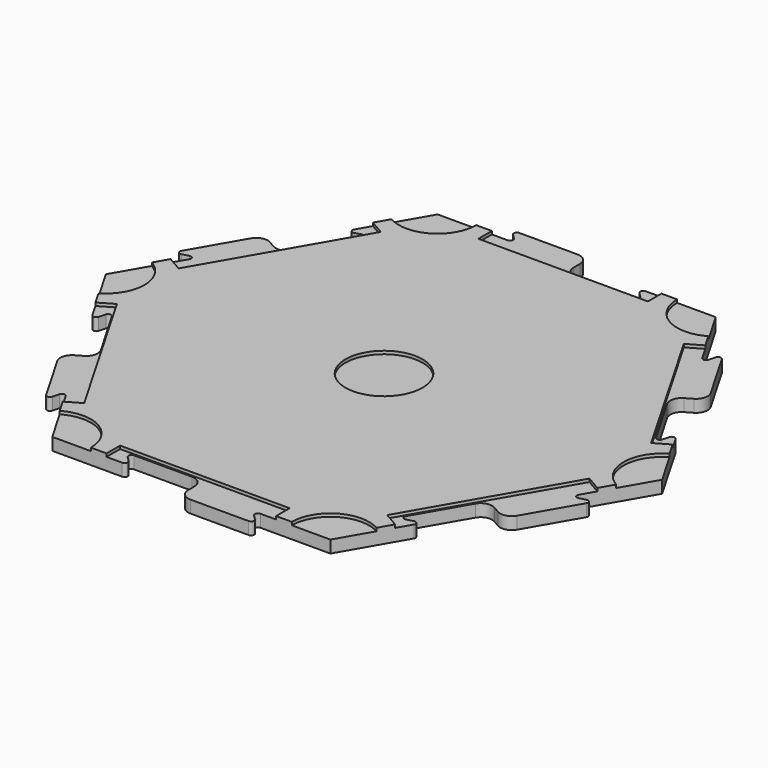
from build123d import *

# Parameters (mm, degrees)
F1_DEPTH = 2.54
F2_COUNT = 6
F4_R     = 6.35
F5_DEPTH = 0.508


# Not quite as in the source:
# - a feature names something its author has since deleted; it is built from what else it names


with BuildPart() as f1:
    # F0 (on Top) → F1 (new body)
    with BuildSketch(Plane.XY):
        with BuildLine():
            Line((11.3864204897, -39.6875), (22.9135888085, -39.6875))
            Line((22.9135888085, -39.6875), (0, 0))
            Line((0, 0), (-22.9135888085, -39.6875))
            Line((-22.9135888085, -39.6875), (-11.3864204897, -39.6875))
            ThreePointArc((-11.3864204897, -39.6875), (-10.9170896872, -39.3739031836), (-11.0272102448, -38.8202897552))
            Line((-11.0272102448, -38.8202897552), (-11.8327897552, -38.0147102448))
            ThreePointArc((-11.8327897552, -38.0147102448), (-11.9429103128, -37.4610968164), (-11.4735795103, -37.1475))
            Line((-11.4735795103, -37.1475), (-1.905, -37.1475))
            ThreePointArc((-1.905, -37.1475), (-0.5579615818, -37.7054615818), (0, -39.0525))
            Line((0, -39.0525), (0, -39.6875))
            Line((0, -39.6875), (11.3864204897, -39.6875))
        make_face()
        with BuildLine():
            ThreePointArc((11.0272102448, -40.5547102448), (10.9170896872, -40.0010968164), (11.3864204897, -39.6875))
            Line((11.3864204897, -39.6875), (0, -39.6875))
            Line((0, -39.6875), (0, -40.3225))
            ThreePointArc((0, -40.3225), (0.5579615818, -41.6695384182), (1.905, -42.2275))
            Line((1.905, -42.2275), (11.4735795103, -42.2275))
            ThreePointArc((11.4735795103, -42.2275), (11.9429103128, -41.9139031836), (11.8327897552, -41.3602897552))
            Line((11.8327897552, -41.3602897552), (11.0272102448, -40.5547102448))
        make_face()
    extrude(amount=F1_DEPTH)


with BuildPart() as f2_1:
    # F2: instance of F1
    add(f1.part.rotate(Axis((0, 0, 1.27), (0, 0, -1)), 1 * 360 / F2_COUNT))


with BuildPart() as f2_2:
    # F2: instance of F1
    add(f1.part.rotate(Axis((0, 0, 1.27), (0, 0, -1)), 2 * 360 / F2_COUNT))


with BuildPart() as f2_3:
    # F2: instance of F1
    add(f1.part.rotate(Axis((0, 0, 1.27), (0, 0, -1)), 3 * 360 / F2_COUNT))


with BuildPart() as f2_4:
    # F2: instance of F1
    add(f1.part.rotate(Axis((0, 0, 1.27), (0, 0, -1)), 4 * 360 / F2_COUNT))


with BuildPart() as f2_5:
    # F2: instance of F1
    add(f1.part.rotate(Axis((0, 0, 1.27), (0, 0, -1)), 5 * 360 / F2_COUNT))


with BuildPart() as f1_1:
    add(f1.part)

    # F3: union F2_1, F2_2, F2_3, F2_4, F2_5
    add(f2_1.part)
    add(f2_2.part)
    add(f2_3.part)
    add(f2_4.part)
    add(f2_5.part)

    # F4 (on face) → F5 (cut)
    with BuildSketch(Plane.XY.offset(2.54)):
        with BuildLine():
            Line((13.97, -36.8935), (-13.97, -36.8935))
            Line((-13.97, -36.8935), (-13.97, -39.6875))
            Line((-13.97, -39.6875), (-11.3864204897, -39.6875))
            ThreePointArc((-11.3864204897, -39.6875), (-10.9170896872, -39.3739031836), (-11.0272102448, -38.8202897552))
            Line((-11.0272102448, -38.8202897552), (-11.8327897552, -38.0147102448))
            ThreePointArc((-11.8327897552, -38.0147102448), (-11.9429103128, -37.4610968164), (-11.4735795103, -37.1475))
            Line((-11.4735795103, -37.1475), (-1.905, -37.1475))
            ThreePointArc((-1.905, -37.1475), (-0.5579615818, -37.7054615818), (0, -39.0525))
            Line((0, -39.0525), (0, -40.3225))
            ThreePointArc((0, -40.3225), (0.5579615818, -41.6695384182), (1.905, -42.2275))
            Line((1.905, -42.2275), (11.4735795103, -42.2275))
            ThreePointArc((11.4735795103, -42.2275), (11.9429103128, -41.9139031836), (11.8327897552, -41.3602897552))
            Line((11.8327897552, -41.3602897552), (11.0272102448, -40.5547102448))
            ThreePointArc((11.0272102448, -40.5547102448), (10.9170896872, -40.0010968164), (11.3864204897, -39.6875))
            Line((11.3864204897, -39.6875), (13.97, -39.6875))
            Line((13.97, -39.6875), (13.97, -36.8935))
        make_face()
        with BuildLine():
            Line((-22.9135888085, -39.6875), (-16.5635888085, -39.6875))
            ThreePointArc((-16.5635888085, -39.6875), (-19.7385888085, -34.188238686), (-26.0885888085, -34.188238686))
            Line((-26.0885888085, -34.188238686), (-22.9135888085, -39.6875))
        make_face()
        with BuildLine():
            ThreePointArc((26.0885888085, -34.188238686), (19.7385888085, -34.188238686), (16.5635888085, -39.6875))
            Line((16.5635888085, -39.6875), (22.9135888085, -39.6875))
            Line((22.9135888085, -39.6875), (26.0885888085, -34.188238686))
        make_face()
        with BuildLine():
            Line((-28.6771729679, -29.7046794022), (-27.3853832127, -31.9421248909))
            Line((-27.3853832127, -31.9421248909), (-24.9657082345, -30.5451248909))
            Line((-24.9657082345, -30.5451248909), (-38.9357082345, -6.3483751091))
            Line((-38.9357082345, -6.3483751091), (-41.3553832127, -7.7453751091))
            Line((-41.3553832127, -7.7453751091), (-40.0635934575, -9.9828205978))
            ThreePointArc((-40.0635934575, -9.9828205978), (-39.5573452468, -10.2324745873), (-39.1329622327, -9.8603006727))
            Line((-39.1329622327, -9.8603006727), (-38.8380996671, -8.7598585968))
            ThreePointArc((-38.8380996671, -8.7598585968), (-38.413716653, -8.3876846821), (-37.9074684422, -8.6373386717))
            Line((-37.9074684422, -8.6373386717), (-33.1231786871, -16.9239716058))
            ThreePointArc((-33.1231786871, -16.9239716058), (-32.9328683822, -18.3695218867), (-33.8204570813, -19.52625))
            Line((-33.8204570813, -19.52625), (-34.9203093441, -20.16125))
            ThreePointArc((-34.9203093441, -20.16125), (-35.8078980432, -21.3179781133), (-35.6175877383, -22.7635283942))
            Line((-35.6175877383, -22.7635283942), (-30.8332979832, -31.0501613283))
            ThreePointArc((-30.8332979832, -31.0501613283), (-30.3270497724, -31.2998153179), (-29.9026667583, -30.9276414032))
            Line((-29.9026667583, -30.9276414032), (-29.6078041927, -29.8271993273))
            ThreePointArc((-29.6078041927, -29.8271993273), (-29.1834211786, -29.4550254127), (-28.6771729679, -29.7046794022))
        make_face()
        with BuildLine():
            Line((24.9657082345, -30.5451248909), (27.3853832127, -31.9421248909))
            Line((27.3853832127, -31.9421248909), (28.6771729679, -29.7046794022))
            ThreePointArc((28.6771729679, -29.7046794022), (28.6402555596, -29.1414285963), (28.1057519878, -28.9599890825))
            Line((28.1057519878, -28.9599890825), (27.005309912, -29.254851648))
            ThreePointArc((27.005309912, -29.254851648), (26.4708063402, -29.0734121342), (26.4338889319, -28.5101613283))
            Line((26.4338889319, -28.5101613283), (31.2181786871, -20.2235283942))
            ThreePointArc((31.2181786871, -20.2235283942), (32.3749068004, -19.3359396951), (33.8204570813, -19.52625))
            Line((33.8204570813, -19.52625), (34.9203093441, -20.16125))
            ThreePointArc((34.9203093441, -20.16125), (36.365859625, -20.3515603049), (37.5225877383, -19.4639716058))
            Line((37.5225877383, -19.4639716058), (42.3068774935, -11.1773386717))
            ThreePointArc((42.3068774935, -11.1773386717), (42.2699600852, -10.6140878658), (41.7354565134, -10.432648352))
            Line((41.7354565134, -10.432648352), (40.6350144376, -10.7275109175))
            ThreePointArc((40.6350144376, -10.7275109175), (40.1005108658, -10.5460714037), (40.0635934575, -9.9828205978))
            Line((40.0635934575, -9.9828205978), (41.3553832127, -7.7453751091))
            Line((41.3553832127, -7.7453751091), (38.9357082345, -6.3483751091))
            Line((38.9357082345, -6.3483751091), (24.9657082345, -30.5451248909))
        make_face()
        with BuildLine():
            Line((-45.8271776169, 0), (-42.6521776169, -5.499261314))
            ThreePointArc((-42.6521776169, -5.499261314), (-40.3279163029, -3.175), (-39.4771776169, 0))
            ThreePointArc((-39.4771776169, 0), (-40.3279163029, 3.175), (-42.6521776169, 5.499261314))
            Line((-42.6521776169, 5.499261314), (-45.8271776169, 0))
        make_face()
        with BuildLine():
            ThreePointArc((42.6521776169, 5.499261314), (39.4771776169, 0), (42.6521776169, -5.499261314))
            Line((42.6521776169, -5.499261314), (45.8271776169, 0))
            Line((45.8271776169, 0), (42.6521776169, 5.499261314))
        make_face()
        with BuildLine():
            Line((-40.0635934575, 9.9828205978), (-41.3553832127, 7.7453751091))
            Line((-41.3553832127, 7.7453751091), (-38.9357082345, 6.3483751091))
            Line((-38.9357082345, 6.3483751091), (-24.9657082345, 30.5451248909))
            Line((-24.9657082345, 30.5451248909), (-27.3853832127, 31.9421248909))
            Line((-27.3853832127, 31.9421248909), (-28.6771729679, 29.7046794022))
            ThreePointArc((-28.6771729679, 29.7046794022), (-28.6402555596, 29.1414285963), (-28.1057519878, 28.9599890825))
            Line((-28.1057519878, 28.9599890825), (-27.005309912, 29.254851648))
            ThreePointArc((-27.005309912, 29.254851648), (-26.4708063402, 29.0734121342), (-26.4338889319, 28.5101613283))
            Line((-26.4338889319, 28.5101613283), (-31.2181786871, 20.2235283942))
            ThreePointArc((-31.2181786871, 20.2235283942), (-32.3749068004, 19.3359396951), (-33.8204570813, 19.52625))
            Line((-33.8204570813, 19.52625), (-34.9203093441, 20.16125))
            ThreePointArc((-34.9203093441, 20.16125), (-36.365859625, 20.3515603049), (-37.5225877383, 19.4639716058))
            Line((-37.5225877383, 19.4639716058), (-42.3068774935, 11.1773386717))
            ThreePointArc((-42.3068774935, 11.1773386717), (-42.2699600852, 10.6140878658), (-41.7354565134, 10.432648352))
            Line((-41.7354565134, 10.432648352), (-40.6350144376, 10.7275109175))
            ThreePointArc((-40.6350144376, 10.7275109175), (-40.1005108658, 10.5460714037), (-40.0635934575, 9.9828205978))
        make_face()
        with BuildLine():
            Line((38.9357082345, 6.3483751091), (41.3553832127, 7.7453751091))
            Line((41.3553832127, 7.7453751091), (40.0635934575, 9.9828205978))
            ThreePointArc((40.0635934575, 9.9828205978), (39.5573452468, 10.2324745873), (39.1329622327, 9.8603006727))
            Line((39.1329622327, 9.8603006727), (38.8380996671, 8.7598585968))
            ThreePointArc((38.8380996671, 8.7598585968), (38.413716653, 8.3876846821), (37.9074684422, 8.6373386717))
            Line((37.9074684422, 8.6373386717), (33.1231786871, 16.9239716058))
            ThreePointArc((33.1231786871, 16.9239716058), (32.9328683822, 18.3695218867), (33.8204570813, 19.52625))
            Line((33.8204570813, 19.52625), (34.9203093441, 20.16125))
            ThreePointArc((34.9203093441, 20.16125), (35.8078980432, 21.3179781133), (35.6175877383, 22.7635283942))
            Line((35.6175877383, 22.7635283942), (30.8332979832, 31.0501613283))
            ThreePointArc((30.8332979832, 31.0501613283), (30.3270497724, 31.2998153179), (29.9026667583, 30.9276414032))
            Line((29.9026667583, 30.9276414032), (29.6078041927, 29.8271993273))
            ThreePointArc((29.6078041927, 29.8271993273), (29.1834211786, 29.4550254127), (28.6771729679, 29.7046794022))
            Line((28.6771729679, 29.7046794022), (27.3853832127, 31.9421248909))
            Line((27.3853832127, 31.9421248909), (24.9657082345, 30.5451248909))
            Line((24.9657082345, 30.5451248909), (38.9357082345, 6.3483751091))
        make_face()
        with BuildLine():
            Line((-22.9135888085, 39.6875), (-26.0885888085, 34.188238686))
            ThreePointArc((-26.0885888085, 34.188238686), (-19.7385888085, 34.188238686), (-16.5635888085, 39.6875))
            Line((-16.5635888085, 39.6875), (-22.9135888085, 39.6875))
        make_face()
        with BuildLine():
            ThreePointArc((16.5635888085, 39.6875), (19.7385888085, 34.188238686), (26.0885888085, 34.188238686))
            Line((26.0885888085, 34.188238686), (22.9135888085, 39.6875))
            Line((22.9135888085, 39.6875), (16.5635888085, 39.6875))
        make_face()
        with BuildLine():
            Line((-11.3864204897, 39.6875), (-13.97, 39.6875))
            Line((-13.97, 39.6875), (-13.97, 36.8935))
            Line((-13.97, 36.8935), (13.97, 36.8935))
            Line((13.97, 36.8935), (13.97, 39.6875))
            Line((13.97, 39.6875), (11.3864204897, 39.6875))
            ThreePointArc((11.3864204897, 39.6875), (10.9170896872, 39.3739031836), (11.0272102448, 38.8202897552))
            Line((11.0272102448, 38.8202897552), (11.8327897552, 38.0147102448))
            ThreePointArc((11.8327897552, 38.0147102448), (11.9429103128, 37.4610968164), (11.4735795103, 37.1475))
            Line((11.4735795103, 37.1475), (1.905, 37.1475))
            ThreePointArc((1.905, 37.1475), (0.5579615818, 37.7054615818), (0, 39.0525))
            Line((0, 39.0525), (0, 40.3225))
            ThreePointArc((0, 40.3225), (-0.5579615818, 41.6695384182), (-1.905, 42.2275))
            Line((-1.905, 42.2275), (-11.4735795103, 42.2275))
            ThreePointArc((-11.4735795103, 42.2275), (-11.9429103128, 41.9139031836), (-11.8327897552, 41.3602897552))
            Line((-11.8327897552, 41.3602897552), (-11.0272102448, 40.5547102448))
            ThreePointArc((-11.0272102448, 40.5547102448), (-10.9170896872, 40.0010968164), (-11.3864204897, 39.6875))
        make_face()
        Circle(F4_R)
    extrude(amount=-F5_DEPTH, mode=Mode.SUBTRACT)


solid = f1_1.part
